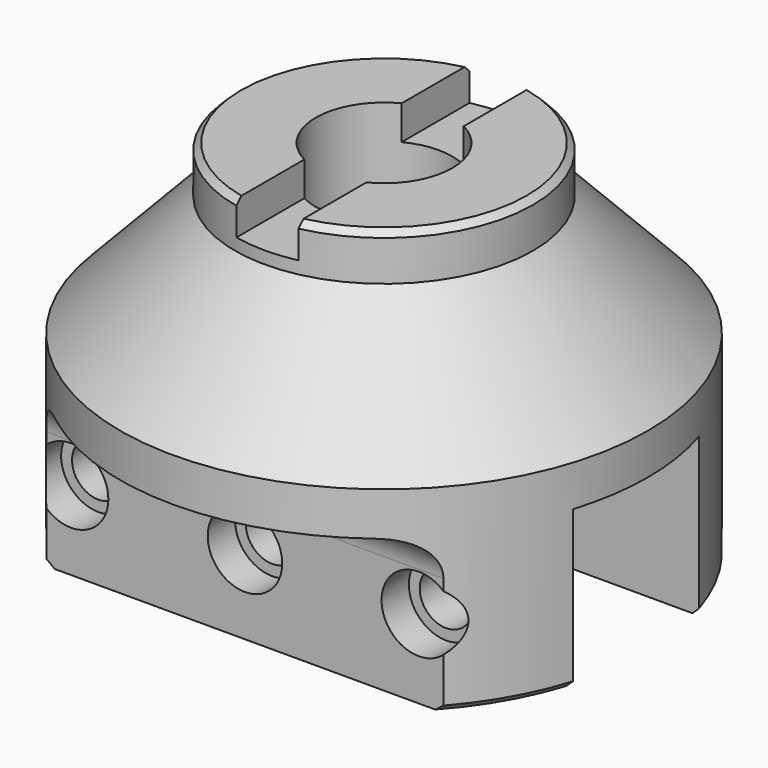
from build123d import *

# Parameters (mm, degrees)
F2_W      = 5.5
F2_H      = 5
F4_W      = 25.4
F4_H      = 25.4
F5_DEPTH  = 50
F6_W      = 10
F6_H      = 5.5
F7_DEPTH  = 25
F8_R      = 4.25
F9_DEPTH  = 50
F10_SIZE  = 1
F12_R     = 6
F13_DEPTH = 25
F15_DEPTH = 40


# Not quite as in the source:
# - a feature names something its author has since deleted; it is built from what else it names


with BuildPart() as f1:
    # F0 (on Front) → F1 (revolve)
    with BuildSketch(Plane.XZ):
        Polygon((0, 59), (0, 0), (42.5, 0), (42.5, 32), (24, 51.5), (24, 59), align=None)
    revolve(axis=Axis((0, 0, 29.5), (0, 0, -1)))

    # F2 (on Front) → F3 (revolve, cut)
    with BuildSketch(Plane.XZ):
        Polygon((5.5, 35), (0, 35), (0, 25), (8.5, 25), (8.5, 35), align=None)
        with Locations((2.75, 37.5)):
            Rectangle(F2_W, F2_H)
        Polygon((11, 59), (0, 59), (0, 40), (5.5, 40), (11, 40), align=None)
    revolve(axis=Axis((0, 0, 30), (0, 0, -1)), mode=Mode.SUBTRACT)

    # F4 (on Right) → F5 (cut, symmetric)
    with BuildSketch(Plane.YZ):
        with Locations((0, 12.7)):
            Rectangle(F4_W, F4_H)
    extrude(amount=F5_DEPTH, both=True, mode=Mode.SUBTRACT)

    # F6 (on Front) → F7 (cut, symmetric)
    with BuildSketch(Plane.XZ):
        with Locations((0, 56.25)):
            Rectangle(F6_W, F6_H)
    extrude(amount=F7_DEPTH, both=True, mode=Mode.SUBTRACT)

    # F8 (on Front) → F9 (cut)
    with BuildSketch(Plane.XZ):
        with Locations((0, 12.7)):
            Circle(F8_R)
        with Locations((28, 12.7)):
            Circle(F8_R)
        with Locations((-28, 12.7)):
            Circle(F8_R)
    extrude(amount=F9_DEPTH, mode=Mode.SUBTRACT)

    # F10
    f10_edges = [f1.edges().sort_by_distance(p)[0] for p in [
        (0, -42.5, 0),
        (0, 42.5, 0),
        (-24, 0, 59),
        (18.654758, -15.099669, 59),
        (18.654758, 15.099669, 59),
    ]]
    chamfer(f10_edges, length=F10_SIZE)

    # F12 (on offset) → F13 (cut)
    with BuildSketch(Plane.XZ.offset(22.5)):
        with Locations((0, 12.7)):
            Circle(F12_R)
        with Locations((-28, 12.7)):
            Circle(F12_R)
        with Locations((28, 12.7)):
            Circle(F12_R)
    extrude(amount=F13_DEPTH, mode=Mode.SUBTRACT)

    # F14 (on Right) → F15 (cut, symmetric)
    with BuildSketch(Plane.YZ):
        with BuildLine():
            Line((-34, 25), (-49.6562516332, 25))
            Line((-49.6562516332, 25), (-49.6562516332, -7.5937491908))
            Line((-49.6562516332, -7.5937491908), (-28, -7.5937491908))
            Line((-28, -7.5937491908), (-28, 19))
            ThreePointArc((-28, 19), (-29.7573593129, 23.2426406871), (-34, 25))
        make_face()
        with BuildLine():
            Line((49.6562516332, -7.5937491908), (49.6562516332, 25))
            Line((49.6562516332, 25), (34, 25))
            ThreePointArc((34, 25), (29.7573593129, 23.2426406871), (28, 19))
            Line((28, 19), (28, -7.5937491908))
            Line((28, -7.5937491908), (49.6562516332, -7.5937491908))
        make_face()
    extrude(amount=F15_DEPTH, both=True, mode=Mode.SUBTRACT)


solid = f1.part
